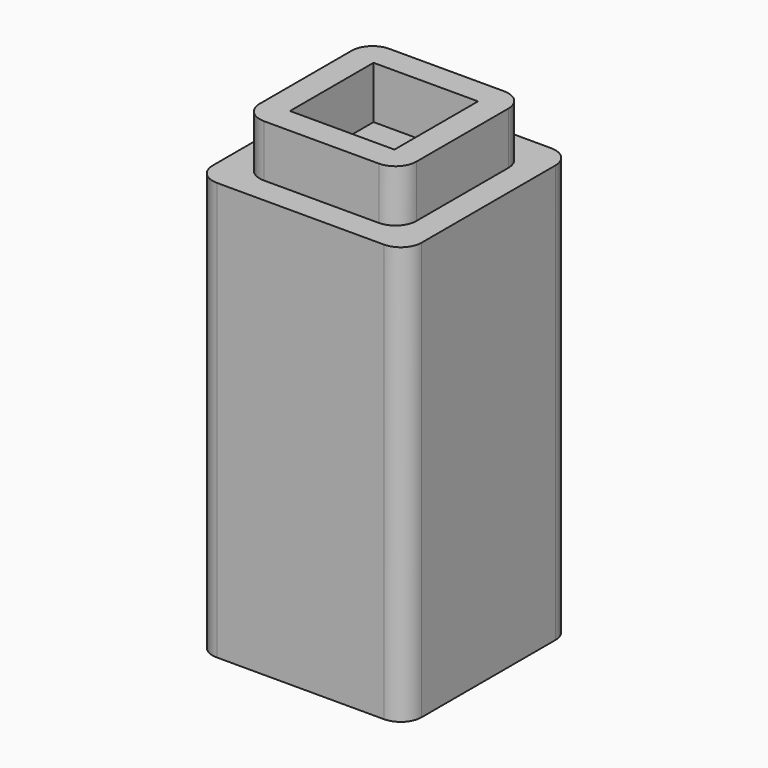
from build123d import *

# Parameters (mm, degrees)
F0_W     = 25.4
F0_H     = 25.4
F1_DEPTH = 50.8
F2_W     = 19.05
F2_H     = 19.05
F3_DEPTH = 44.45
F4_W     = 19.05
F4_H     = 19.05
F4_W_2   = 12.7
F4_H_2   = 12.7
F5_DEPTH = 6.35
F6_R     = 2.54


# Not quite as in the source:
# - a feature names something its author has since deleted; it is built from what else it names


with BuildPart() as f1:
    # F0 (on Top) → F1 (new body)
    with BuildSketch(Plane.XY):
        with Locations((12.7, -12.7)):
            Rectangle(F0_W, F0_H)
    extrude(amount=F1_DEPTH)

    # F2 (on face) → F3 (cut)
    with BuildSketch(Plane(origin=(0, 0, 0), x_dir=(1, 0, 0), z_dir=(0, 0, -1))):
        with Locations((12.7, 12.7)):
            Rectangle(F2_W, F2_H)
    extrude(amount=-F3_DEPTH, mode=Mode.SUBTRACT)

    # F4 (on face) → F5 (join)
    with BuildSketch(Plane.XY.offset(50.8)):
        with Locations((12.7, -12.7)):
            Rectangle(F4_W, F4_H)
        with Locations((12.7, -12.7)):
            Rectangle(F4_W_2, F4_H_2, mode=Mode.SUBTRACT)
    extrude(amount=F5_DEPTH)

    # F6
    f6_edges = [f1.edges().sort_by_distance(p)[0] for p in [
        (0, 0, 25.4),
        (0, -25.4, 25.4),
        (25.4, 0, 25.4),
        (3.175, -3.175, 53.975),
        (3.175, -22.225, 53.975),
        (22.225, -3.175, 53.975),
        (22.225, -22.225, 53.975),
        (25.4, -25.4, 25.4),
    ]]
    fillet(f6_edges, radius=F6_R)


solid = f1.part
